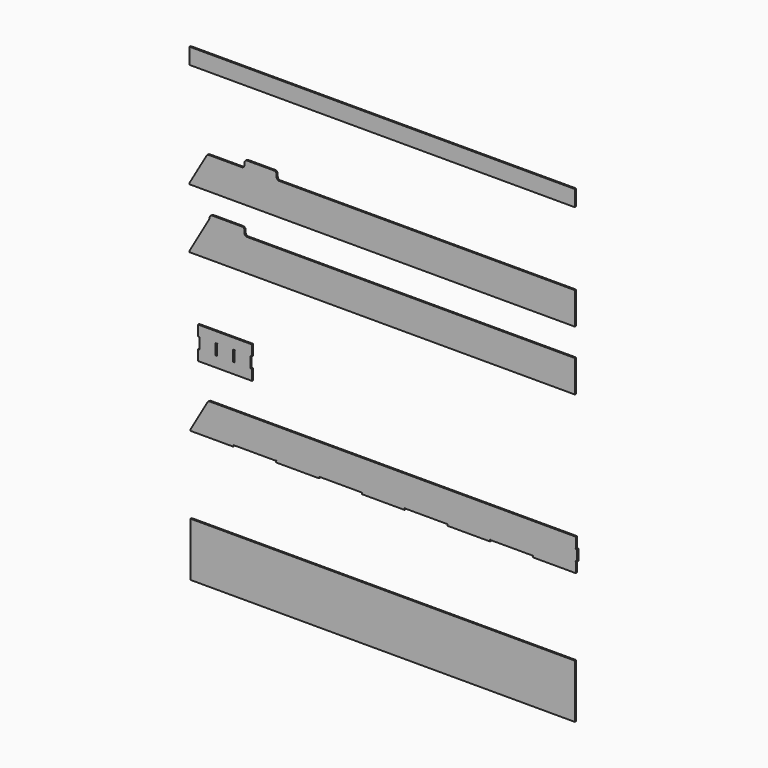
from build123d import *

# Parameters (mm, degrees)
F1_W      = 914.4
F1_H      = 38.1
F2_DEPTH  = 3.4163
F4_DEPTH  = 3.4163
F6_DEPTH  = 3.4036
F8_DEPTH  = 3.4163
F10_DEPTH = 3.4163
F11_W     = 912.2229164778
F11_H     = 127.9652
F12_DEPTH = 3.429


# Not quite as in the source:
# - ends of sketch curves that miss each other by under 0.0002 mm in the source are joined


with BuildPart() as f2:
    # F1 (on Front) → F2 (new body)
    with BuildSketch(Plane.XZ):
        with Locations((12.759034133, -162.508072567)):
            Rectangle(F1_W, F1_H)
    extrude(amount=F2_DEPTH)


with BuildPart() as f4:
    # F3 (on Front) → F4 (new body)
    with BuildSketch(Plane.XZ):
        with BuildLine():
            Line((-320.590565867, -354.8278894318), (-398.7531028701, -354.8278894318))
            ThreePointArc((-398.7531028701, -354.8278894318), (-401.9281028701, -355.6786281177), (-404.2523641841, -358.0028894318))
            Line((-404.2523641841, -358.0028894318), (-444.440965867, -427.6115894318))
            Line((-444.440965867, -427.6115894318), (-444.440965867, -431.0278894318))
            Line((-444.440965867, -431.0278894318), (469.959034133, -431.0278894318))
            Line((469.959034133, -431.0278894318), (469.959034133, -354.8278894318))
            Line((469.959034133, -354.8278894318), (-231.690565867, -354.8278894318))
            ThreePointArc((-231.690565867, -354.8278894318), (-236.1806939276, -352.9680174923), (-238.040565867, -348.4778894318))
            Line((-238.040565867, -348.4778894318), (-238.040565867, -343.3978894318))
            ThreePointArc((-238.040565867, -343.3978894318), (-239.9004378065, -338.9077613712), (-244.390565867, -337.0478894318))
            Line((-244.390565867, -337.0478894318), (-307.890565867, -337.0478894318))
            ThreePointArc((-307.890565867, -337.0478894318), (-312.3806939276, -338.9077613712), (-314.240565867, -343.3978894318))
            Line((-314.240565867, -343.3978894318), (-314.240565867, -348.4778894318))
            ThreePointArc((-314.240565867, -348.4778894318), (-316.1004378065, -352.9680174923), (-320.590565867, -354.8278894318))
        make_face()
    extrude(amount=F4_DEPTH)


with BuildPart() as f6:
    # F5 (on Front) → F6 (new body)
    with BuildSketch(Plane.XZ):
        with BuildLine():
            Line((469.959034133, -572.8818325169), (469.959034133, -496.6818325169))
            Line((469.959034133, -496.6818325169), (-307.8807011454, -496.6818325169))
            ThreePointArc((-307.8807011454, -496.6818325169), (-312.370829206, -494.8219605774), (-314.2307011454, -490.3318325169))
            Line((-314.2307011454, -490.3318325169), (-314.2307011454, -485.2518325169))
            ThreePointArc((-314.2307011454, -485.2518325169), (-316.0905730849, -480.7617044564), (-320.5807011454, -478.9018325169))
            Line((-320.5807011454, -478.9018325169), (-390.4307011454, -478.9018325169))
            ThreePointArc((-390.4307011454, -478.9018325169), (-394.9141460418, -480.7550312247), (-396.780673052, -485.2329437416))
            ThreePointArc((-396.780673052, -485.2329437416), (-396.9995232777, -486.8666766847), (-397.6314398314, -488.389055145))
            Line((-397.6314398314, -488.389055145), (-444.440965867, -569.4655325169))
            Line((-444.440965867, -569.4655325169), (-444.440965867, -572.8818325169))
            Line((-444.440965867, -572.8818325169), (469.959034133, -572.8818325169))
        make_face()
    extrude(amount=F6_DEPTH)


with BuildPart() as f8:
    # F7 (on Front) → F8 (new body)
    with BuildSketch(Plane.XZ):
        with BuildLine():
            Line((-296.4323394764, -717.5106746197), (-424.3975394764, -717.5106746197))
            Line((-424.3975394764, -717.5106746197), (-424.3975394764, -742.7836746197))
            Line((-424.3975394764, -742.7836746197), (-421.4892394764, -742.7836746197))
            ThreePointArc((-421.4892394764, -742.7836746197), (-420.6220292316, -742.4244643748), (-420.9812394764, -743.2916746197))
            Line((-420.9812394764, -743.2916746197), (-420.9812394764, -755.6106746197))
            Line((-420.9812394764, -755.6106746197), (-420.9812394764, -767.9296746197))
            ThreePointArc((-420.9812394764, -767.9296746197), (-420.6220292316, -768.7968848645), (-421.4892394764, -768.4376746197))
            Line((-421.4892394764, -768.4376746197), (-424.3975394764, -768.4376746197))
            Line((-424.3975394764, -768.4376746197), (-424.3975394764, -793.7106746197))
            Line((-424.3975394764, -793.7106746197), (-296.4323394764, -793.7106746197))
            Line((-296.4323394764, -793.7106746197), (-296.4323394764, -768.4376746197))
            Line((-296.4323394764, -768.4376746197), (-299.3406394764, -768.4376746197))
            ThreePointArc((-299.3406394764, -768.4376746197), (-300.2078497213, -768.7968848645), (-299.8486394764, -767.9296746197))
            Line((-299.8486394764, -767.9296746197), (-299.8486394764, -755.6106746197))
            Line((-299.8486394764, -755.6106746197), (-299.8486394764, -743.2916746197))
            ThreePointArc((-299.8486394764, -743.2916746197), (-300.2078497213, -742.4244643748), (-299.3406394764, -742.7836746197))
            Line((-299.3406394764, -742.7836746197), (-296.4323394764, -742.7836746197))
            Line((-296.4323394764, -742.7836746197), (-296.4323394764, -717.5106746197))
        make_face()
        with BuildLine():
            Line((-383.0082394764, -755.6106746197), (-383.0082394764, -743.2916746197))
            ThreePointArc((-383.0082394764, -743.2916746197), (-383.3674497213, -742.4244643748), (-382.5002394764, -742.7836746197))
            Line((-382.5002394764, -742.7836746197), (-379.8205394764, -742.7836746197))
            ThreePointArc((-379.8205394764, -742.7836746197), (-378.9533292316, -742.4244643748), (-379.3125394764, -743.2916746197))
            Line((-379.3125394764, -743.2916746197), (-379.3125394764, -755.6106746197))
            Line((-379.3125394764, -755.6106746197), (-379.3125394764, -767.9296746197))
            ThreePointArc((-379.3125394764, -767.9296746197), (-378.9533292316, -768.7968848645), (-379.8205394764, -768.4376746197))
            Line((-379.8205394764, -768.4376746197), (-382.5002394764, -768.4376746197))
            ThreePointArc((-382.5002394764, -768.4376746197), (-383.3674497213, -768.7968848645), (-383.0082394764, -767.9296746197))
            Line((-383.0082394764, -767.9296746197), (-383.0082394764, -755.6106746197))
        make_face(mode=Mode.SUBTRACT)
        with BuildLine():
            Line((-341.5173394764, -755.6106746197), (-341.5173394764, -743.2916746197))
            ThreePointArc((-341.5173394764, -743.2916746197), (-341.8765497213, -742.4244643748), (-341.0093394764, -742.7836746197))
            Line((-341.0093394764, -742.7836746197), (-338.3296394764, -742.7836746197))
            ThreePointArc((-338.3296394764, -742.7836746197), (-337.4624292316, -742.4244643748), (-337.8216394764, -743.2916746197))
            Line((-337.8216394764, -743.2916746197), (-337.8216394764, -755.6106746197))
            Line((-337.8216394764, -755.6106746197), (-337.8216394764, -767.9296746197))
            ThreePointArc((-337.8216394764, -767.9296746197), (-337.4624292316, -768.7968848645), (-338.3296394764, -768.4376746197))
            Line((-338.3296394764, -768.4376746197), (-341.0093394764, -768.4376746197))
            ThreePointArc((-341.0093394764, -768.4376746197), (-341.8765497213, -768.7968848645), (-341.5173394764, -767.9296746197))
            Line((-341.5173394764, -767.9296746197), (-341.5173394764, -755.6106746197))
        make_face(mode=Mode.SUBTRACT)
    extrude(amount=F8_DEPTH)


with BuildPart() as f10:
    # F9 (on Front) → F10 (new body)
    with BuildSketch(Plane.XZ):
        with BuildLine():
            Line((-442.1973738139, -942.08762847), (-442.1973738139, -945.50392847))
            Line((-442.1973738139, -945.50392847), (-340.5973738139, -945.50392847))
            Line((-340.5973738139, -945.50392847), (-340.5973738139, -942.59562847))
            ThreePointArc((-340.5973738139, -942.59562847), (-340.9565840588, -941.7284182251), (-340.0893738139, -942.08762847))
            Line((-340.0893738139, -942.08762847), (-239.5053738139, -942.08762847))
            ThreePointArc((-239.5053738139, -942.08762847), (-238.6381635691, -941.7284182251), (-238.9973738139, -942.59562847))
            Line((-238.9973738139, -942.59562847), (-238.9973738139, -945.50392847))
            Line((-238.9973738139, -945.50392847), (-137.3973738139, -945.50392847))
            Line((-137.3973738139, -945.50392847), (-137.3973738139, -942.59562847))
            ThreePointArc((-137.3973738139, -942.59562847), (-137.7565840588, -941.7284182251), (-136.8893738139, -942.08762847))
            Line((-136.8893738139, -942.08762847), (-36.3053738139, -942.08762847))
            ThreePointArc((-36.3053738139, -942.08762847), (-35.4381635691, -941.7284182251), (-35.7973738139, -942.59562847))
            Line((-35.7973738139, -942.59562847), (-35.7973738139, -945.50392847))
            Line((-35.7973738139, -945.50392847), (65.8026261861, -945.50392847))
            Line((65.8026261861, -945.50392847), (65.8026261861, -942.59562847))
            ThreePointArc((65.8026261861, -942.59562847), (65.4434159412, -941.7284182251), (66.3106261861, -942.08762847))
            Line((66.3106261861, -942.08762847), (166.8946261861, -942.08762847))
            ThreePointArc((166.8946261861, -942.08762847), (167.7618364309, -941.7284182251), (167.4026261861, -942.59562847))
            Line((167.4026261861, -942.59562847), (167.4026261861, -945.50392847))
            Line((167.4026261861, -945.50392847), (269.0026261861, -945.50392847))
            Line((269.0026261861, -945.50392847), (269.0026261861, -942.59562847))
            ThreePointArc((269.0026261861, -942.59562847), (268.6434159412, -941.7284182251), (269.5106261861, -942.08762847))
            Line((269.5106261861, -942.08762847), (370.0946261861, -942.08762847))
            ThreePointArc((370.0946261861, -942.08762847), (370.9618364309, -941.7284182251), (370.6026261861, -942.59562847))
            Line((370.6026261861, -942.59562847), (370.6026261861, -945.50392847))
            Line((370.6026261861, -945.50392847), (472.2026261861, -945.50392847))
            Line((472.2026261861, -945.50392847), (472.2026261861, -920.61192847))
            ThreePointArc((472.2026261861, -920.61192847), (471.8434159412, -919.7447182251), (472.7106261861, -920.10392847))
            Line((472.7106261861, -920.10392847), (475.6189261861, -920.10392847))
            Line((475.6189261861, -920.10392847), (475.6189261861, -907.40392847))
            Line((475.6189261861, -907.40392847), (475.6189261861, -894.70392847))
            Line((475.6189261861, -894.70392847), (472.7106261861, -894.70392847))
            ThreePointArc((472.7106261861, -894.70392847), (471.8434159412, -895.0631387148), (472.2026261861, -894.19592847))
            Line((472.2026261861, -894.19592847), (472.2026261861, -869.30392847))
            Line((472.2026261861, -869.30392847), (-396.5095108169, -869.30392847))
            ThreePointArc((-396.5095108169, -869.30392847), (-399.6845108169, -870.1546671559), (-402.008772131, -872.47892847))
            Line((-402.008772131, -872.47892847), (-442.1973738139, -942.08762847))
        make_face()
    extrude(amount=F10_DEPTH)


with BuildPart() as f12:
    # F11 (on Front) → F12 (new body)
    with BuildSketch(Plane.XZ):
        with Locations((13.914084425, -1193.0309593414)):
            Rectangle(F11_W, F11_H)
    extrude(amount=F12_DEPTH)


solid = Compound([f2.part, f4.part, f6.part, f8.part, f10.part, f12.part])
